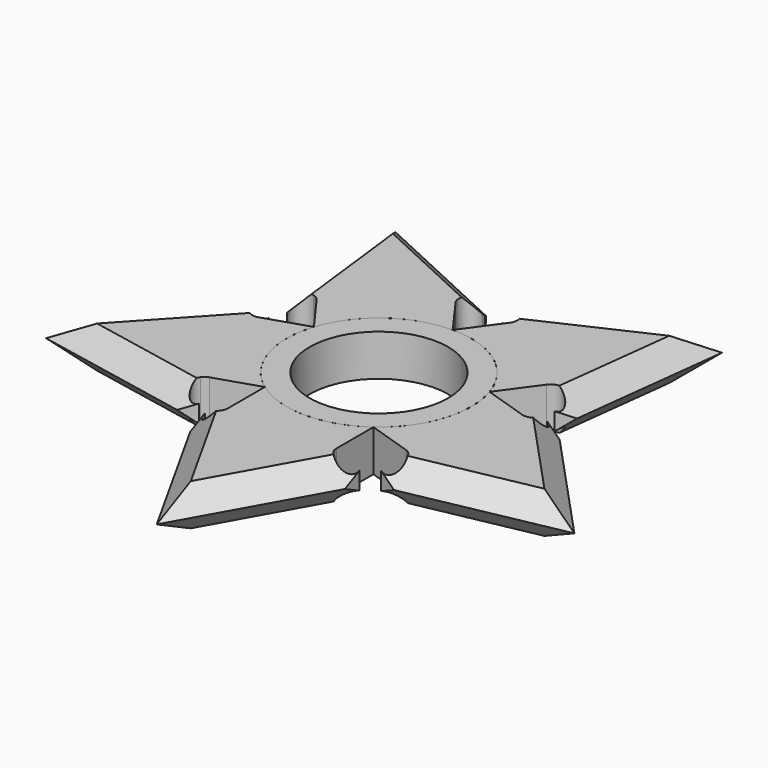
from build123d import *

# Parameters (mm, degrees)
F0_R        = 20
F0_R_2      = 15
F1_DEPTH    = 9
F3_DEPTH    = 9
F4_SIZE     = 5
F5_T1_DEPTH = 60.0789260262
F5_T3_DEPTH = 60.0789260262
F6_COUNT    = 5


# Not quite as in the source:
# - a fillet or chamfer that OpenCascade refuses, or shapes differently, is made with other operations: its cross-section is extruded or revolved along the edge and cut away or added


with BuildPart() as f1:
    # F0 (on Top) → F1 (new body)
    with BuildSketch(Plane.XY):
        Circle(F0_R)
        Circle(F0_R_2, mode=Mode.SUBTRACT)
    extrude(amount=F1_DEPTH)


with BuildPart() as f3:
    # F2 (on face) → F3 (new body)
    with BuildSketch(Plane(origin=(0, 0, 0), x_dir=(1, 0, 0), z_dir=(0, 0, -1))):
        with BuildLine():
            ThreePointArc((19.0211303259, -6.1803398875), (11.7557050458, -16.1803398875), (0, -20))
            Line((0, -20), (5.8778525229, -28.0901699437))
            ThreePointArc((5.8778525229, -28.0901699437), (6.2329513277, -28.7870905885), (6.355310037, -29.5596330745))
            ThreePointArc((6.355310037, -29.5596330745), (4.6278525229, -31.9372743652), (1.832767551, -31.0290962052))
            Line((1.832767551, -31.0290962052), (4.7716938125, -35.0741811771))
            Line((4.7716938125, -35.0741811771), (35.9609015161, -49.4959346906))
            Line((35.9609015161, -49.4959346906), (31.8829940822, -15.3766685417))
            Line((31.8829940822, -15.3766685417), (28.9440678207, -11.3315835698))
            ThreePointArc((28.9440678207, -11.3315835698), (29.2991666255, -12.0285042146), (29.4215253348, -12.8010467005))
            ThreePointArc((29.4215253348, -12.8010467005), (27.6940678207, -15.1786879913), (24.8989828488, -14.2705098312))
            Line((24.8989828488, -14.2705098312), (19.0211303259, -6.1803398875))
        make_face()
    extrude(amount=-F3_DEPTH)

    # F4
    f4_edges = [f3.edges().sort_by_distance(p)[0] for p in [
        (33.921948, 32.436302, 9),
        (20.366298, 42.285058, 9),
    ]]
    chamfer(f4_edges, length=F4_SIZE)

    # F5: chamfer of 5 on 2 edges, made by hand

    # F5_s2 → F5_t1 (cut)
    with BuildSketch(Plane(origin=(7.8648277039, 65.8038844656, 0), x_dir=(0, 0, 1), z_dir=(-0.1186745831, -0.9929332018, 0))):
        Polygon((0, -24.8328636701), (5, -29.8328636701), (0, -29.8328636701), align=None)
    extrude(amount=F5_T1_DEPTH, mode=Mode.SUBTRACT)

    # F5_s4 → F5_t3 (cut)
    with BuildSketch(Plane(origin=(5.6214217229, 2.5993208694, 0), x_dir=(0, 0, 1), z_dir=(0.9076631289, 0.4196994692, 0))):
        Polygon((0, -24.8328636701), (5, -29.8328636701), (0, -29.8328636701), align=None)
    extrude(amount=F5_T3_DEPTH, mode=Mode.SUBTRACT)


with BuildPart() as f6_1:
    # F6: instance of F3
    add(f3.part.rotate(Axis((0, 0, 9), (0, 0, 1)), 1 * 360 / F6_COUNT))


with BuildPart() as f6_2:
    # F6: instance of F3
    add(f3.part.rotate(Axis((0, 0, 9), (0, 0, 1)), 2 * 360 / F6_COUNT))


with BuildPart() as f6_3:
    # F6: instance of F3
    add(f3.part.rotate(Axis((0, 0, 9), (0, 0, 1)), 3 * 360 / F6_COUNT))


with BuildPart() as f6_4:
    # F6: instance of F3
    add(f3.part.rotate(Axis((0, 0, 9), (0, 0, 1)), 4 * 360 / F6_COUNT))


solid = Compound([f1.part, f3.part, f6_1.part, f6_2.part, f6_3.part, f6_4.part])
